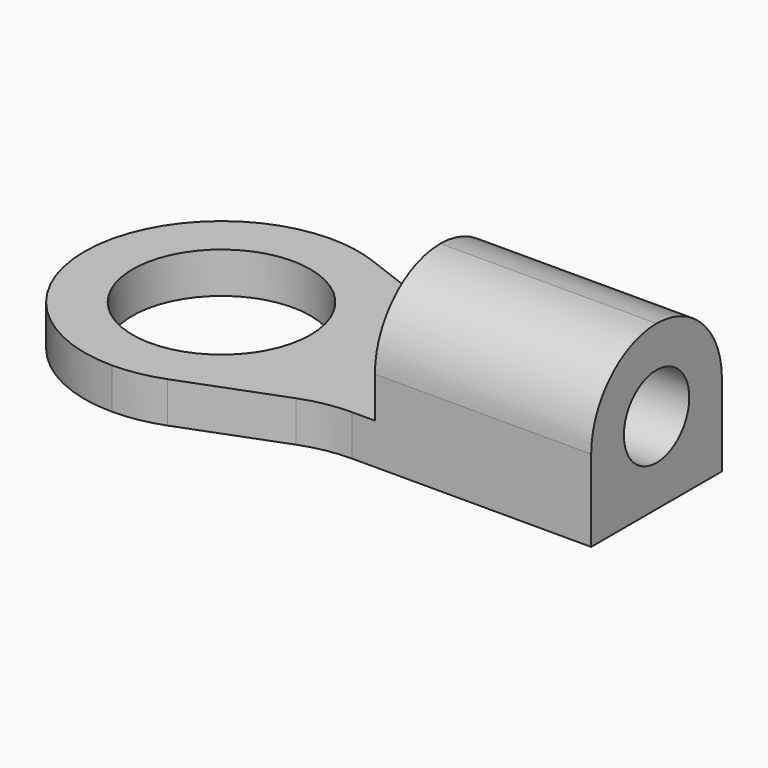
from build123d import *

# Parameters (mm, degrees)
F0_R     = 1.85
F1_DEPTH = 0.85
F2_W     = 4.5
F2_H     = 3.4
F3_DEPTH = 2.55
F4_R     = 1.69999
F5_R     = 0.85
F6_DEPTH = 25


# Not quite as in the source:
# - a fillet or chamfer is up to 0.001 mm smaller than in the source, because OpenCascade refuses the exact size


with BuildPart() as f1:
    # F0 (on Top) → F1 (new body)
    with BuildSketch(Plane.XY):
        with BuildLine():
            Line((6.9231632929, 1.15), (11.9, 1.15))
            Line((11.9, 1.15), (11.9, 4.55))
            Line((11.9, 4.55), (6.9231632929, 4.55))
            ThreePointArc((6.9231632929, 4.55), (6.408597702, 4.5968370984), (5.9109449246, 4.7358089455))
            Line((5.9109449246, 4.7358089455), (3.8622183683, 5.5141910545))
            ThreePointArc((3.8622183683, 5.5141910545), (3.3645655909, 5.6531629016), (2.85, 5.7))
            ThreePointArc((2.85, 5.7), (0.8347456736, 4.8652543264), (0, 2.85))
            ThreePointArc((0, 2.85), (0.8347456736, 0.8347456736), (2.85, 0))
            ThreePointArc((2.85, 0), (3.3645655909, 0.0468370984), (3.8622183683, 0.1858089455))
            Line((3.8622183683, 0.1858089455), (5.9109449246, 0.9641910545))
            ThreePointArc((5.9109449246, 0.9641910545), (6.408597702, 1.1031629016), (6.9231632929, 1.15))
        make_face()
        with Locations((2.85, 2.85)):
            Circle(F0_R, mode=Mode.SUBTRACT)
    extrude(amount=F1_DEPTH)

    # F2 (on face) → F3 (join)
    with BuildSketch(Plane.XY.offset(0.85)):
        with Locations((9.65, 2.85)):
            Rectangle(F2_W, F2_H)
    extrude(amount=F3_DEPTH)

    # F4 (radius 1.7 in the source; OpenCascade refuses exactly that, so slightly less here)
    f4_edges = [f1.edges().sort_by_distance(p)[0] for p in [
        (9.65, 4.55, 3.4),
        (9.65, 1.15, 3.4),
    ]]
    fillet(f4_edges, radius=F4_R)

    # F5 (on face) → F6 (cut)
    with BuildSketch(Plane.YZ.offset(11.9)):
        with Locations((2.85, 1.7)):
            Circle(F5_R)
    extrude(amount=-F6_DEPTH, mode=Mode.SUBTRACT)


solid = f1.part
